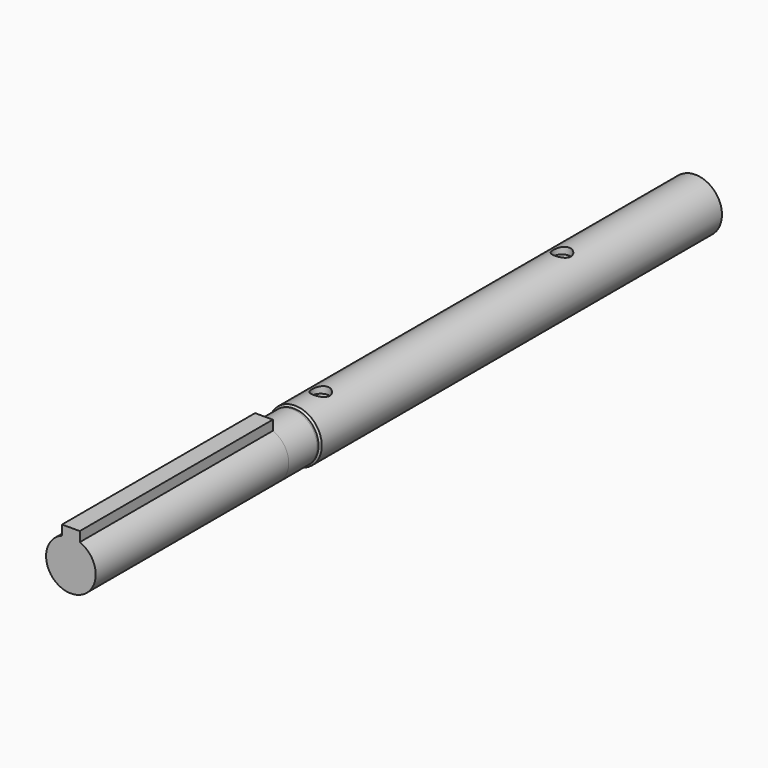
from build123d import *

# Parameters (mm, degrees)
F1_DEPTH    = 34
F2_R        = 7
F3_DEPTH    = 10
F4_R        = 7.5
F5_DEPTH    = 142
F7_R        = 2.5
F8_DEPTH    = 2
F9_S5_R     = 7
F9_T6_DEPTH = 12


# Not quite as in the source:
# - a fillet or chamfer that OpenCascade refuses, or shapes differently, is made with other operations: its cross-section is extruded or revolved along the edge and cut away or added
# - after a boolean that leaves OpenCascade's solid faulty, fix() repairs it


with BuildPart() as f1:
    # F0 (on Front) → F1 (new body, symmetric)
    with BuildSketch(Plane.XZ):
        with BuildLine():
            Line((-2.5, 9.3003484153), (-2.5, 6.5383484153))
            ThreePointArc((-2.5, 6.5383484153), (0, -7), (2.5, 6.5383484153))
            Line((2.5, 6.5383484153), (2.5, 9.3003484153))
            Line((2.5, 9.3003484153), (-2.5, 9.3003484153))
        make_face()
    extrude(amount=F1_DEPTH, both=True)

    # F2 (on face) → F3 (join)
    with BuildSketch(Plane(origin=(0, 34, 0), x_dir=(-1, 0, 0), z_dir=(0, 1, 0))):
        Circle(F2_R)
    extrude(amount=F3_DEPTH)

    # F4 (on face) → F5 (join)
    with BuildSketch(Plane(origin=(0, 44, 0), x_dir=(-1, 0, 0), z_dir=(0, 1, 0))):
        Circle(F4_R)
    extrude(amount=F5_DEPTH)

    add(f1.part.fix(), mode=Mode.REPLACE)

    # F7 (on offset) → F8 (cut)
    with BuildSketch(Plane.XY.offset(7.5)):
        with Locations((0, 54)):
            Circle(F7_R)
        with Locations((0, 139)):
            Circle(F7_R)
    extrude(amount=-F8_DEPTH, mode=Mode.SUBTRACT)

    # F9: chamfer of 1 on 1 edges, made by hand


with BuildPart() as f9_tool2:
    # F9_s3 → F9_t4 (revolve)
    with BuildSketch(Plane.XY):
        Polygon((-7.5, 45), (-6.5, 44), (-7.5, 44), align=None)
    revolve(axis=Axis((0, 44, 0), (0, 1, 0)))

    # F9_s5 → F9_t6 (cut, symmetric)
    with BuildSketch(Plane.XZ.offset(-44.5)):
        Circle(F9_S5_R)
    extrude(amount=F9_T6_DEPTH, both=True, mode=Mode.SUBTRACT)


with BuildPart() as f1_1:
    add(f1.part)

    # F9_t1: cut F9_tool2
    add(f9_tool2.part, mode=Mode.SUBTRACT)


solid = f1_1.part
